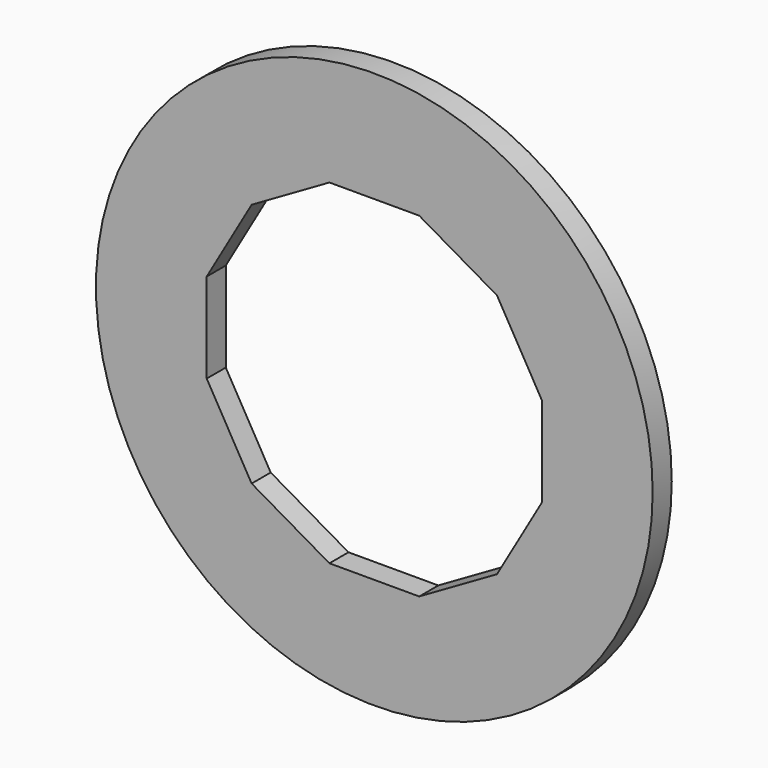
from build123d import *

# Parameters (mm, degrees)
F0_R     = 70
F1_DEPTH = 3


# Not quite as in the source:
# - a feature of the source that left no trace in its solid (it failed there, or was rolled back) is left out


with BuildPart() as f1:
    # F0 (on Front) → F1 (new body, symmetric)
    with BuildSketch(Plane.XZ):
        Circle(F0_R)
        Polygon((-30.855941539, 30.855941539), (-11.294058461, 42.15), (11.294058461, 42.15), (30.855941539, 30.855941539), (42.15, 11.294058461), (42.15, -11.294058461), (30.855941539, -30.855941539), (11.294058461, -42.15), (-11.294058461, -42.15), (-30.855941539, -30.855941539), (-42.15, -11.294058461), (-42.15, 11.294058461), align=None, mode=Mode.SUBTRACT)
    extrude(amount=F1_DEPTH, both=True)


solid = f1.part
